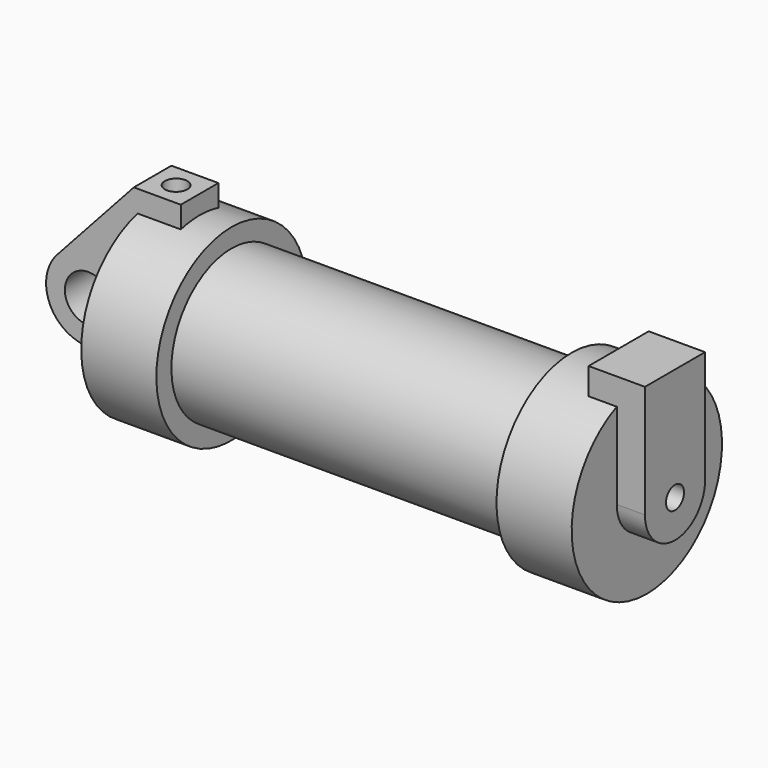
from build123d import *

# Parameters (mm, degrees)
F0_R     = 3.175
F0_W     = 5.842
F0_H     = 12.7
F2_DEPTH = 3.175
F4_R     = 1.524
F5_DEPTH = 3.81
F7_R     = 1.524
F9_DEPTH = 17.78


# Not quite as in the source:
# - the program builds the solid bodies; features that only make, move or delete a surface that nothing else refers to are left out


with BuildPart() as f1:
    # F0 (on Front) → F1 (revolve)
    with BuildSketch(Plane.XZ):
        Polygon((5.842, 12.7), (5.842, 0), (66.294, 0), (66.294, 12.7), (56.134, 12.7), (56.134, 10.16), (10.16, 10.16), (10.16, 12.7), align=None)
    revolve(axis=Axis((33.147, 0, 0), (-1, 0, 0)))

    # F0 (on Front) → F2 (join, symmetric)
    with BuildSketch(Plane.XZ):
        with BuildLine():
            Line((5.842, 0), (0, 0))
            Line((0, 0), (-0.9398, 0))
            ThreePointArc((-0.9398, 0), (-3.1957909266, -4.5493385486), (-8.1826630726, -5.5069827884))
            Line((-8.1826630726, -5.5069827884), (5.842, -9.398))
            Line((5.842, -9.398), (5.842, 0))
        make_face()
        with BuildLine():
            ThreePointArc((-8.1826630726, -5.5069827884), (-3.1957909266, -4.5493385486), (-0.9398, 0))
            ThreePointArc((-0.9398, 0), (-4.5919612295, 5.3297205562), (-10.8806298187, 3.8475430269))
            ThreePointArc((-10.8806298187, 3.8475430269), (-12.1459778134, -1.5837270034), (-8.1826630726, -5.5069827884))
        make_face()
        with Locations((-6.6548, 0)):
            Circle(F0_R, mode=Mode.SUBTRACT)
        with BuildLine():
            Line((-0.9398, 0), (0, 0))
            Line((0, 0), (0, 12.7))
            Line((0, 12.7), (5.842, 12.7))
            Line((5.842, 12.7), (5.842, 15.24))
            Line((5.842, 15.24), (-0.508, 15.24))
            Line((-0.508, 15.24), (-10.8806298187, 3.8475430269))
            ThreePointArc((-10.8806298187, 3.8475430269), (-4.5919612295, 5.3297205562), (-0.9398, 0))
        make_face()
        with Locations((2.921, 6.35)):
            Rectangle(F0_W, F0_H)
    extrude(amount=F2_DEPTH, both=True)

    # F0 (on Front) → F3 (revolve)
    with BuildSketch(Plane.XZ):
        with Locations((2.921, 6.35)):
            Rectangle(F0_W, F0_H)
    revolve(axis=Axis((33.147, 0, 0), (-1, 0, 0)))

    # F4 (on face) → F5 (join, symmetric)
    with BuildSketch(Plane.YZ.offset(66.294)):
        with BuildLine():
            ThreePointArc((-5.08, 0), (0, -5.08), (5.08, 0))
            ThreePointArc((5.08, 0), (0, 5.08), (-5.08, 0))
        make_face()
        Circle(F4_R, mode=Mode.SUBTRACT)
        with BuildLine():
            ThreePointArc((-5.08, 0), (0, 5.08), (5.08, 0))
            Line((5.08, 0), (5.08, 11.6397422652))
            ThreePointArc((5.08, 11.6397422652), (0, 12.7), (-5.08, 11.6397422652))
            Line((-5.08, 11.6397422652), (-5.08, 0))
        make_face()
        with BuildLine():
            ThreePointArc((-5.08, 11.6397422652), (0, 12.7), (5.08, 11.6397422652))
            Line((5.08, 11.6397422652), (5.08, 15.24))
            Line((5.08, 15.24), (-5.08, 15.24))
            Line((-5.08, 15.24), (-5.08, 11.6397422652))
        make_face()
    extrude(amount=F5_DEPTH, both=True)

    # F7 (on face) → F9 (cut)
    with BuildSketch(Plane.XY.offset(15.24)):
        with Locations((2.667, 0)):
            Circle(F7_R)
    extrude(amount=-F9_DEPTH, mode=Mode.SUBTRACT)


solid = f1.part
